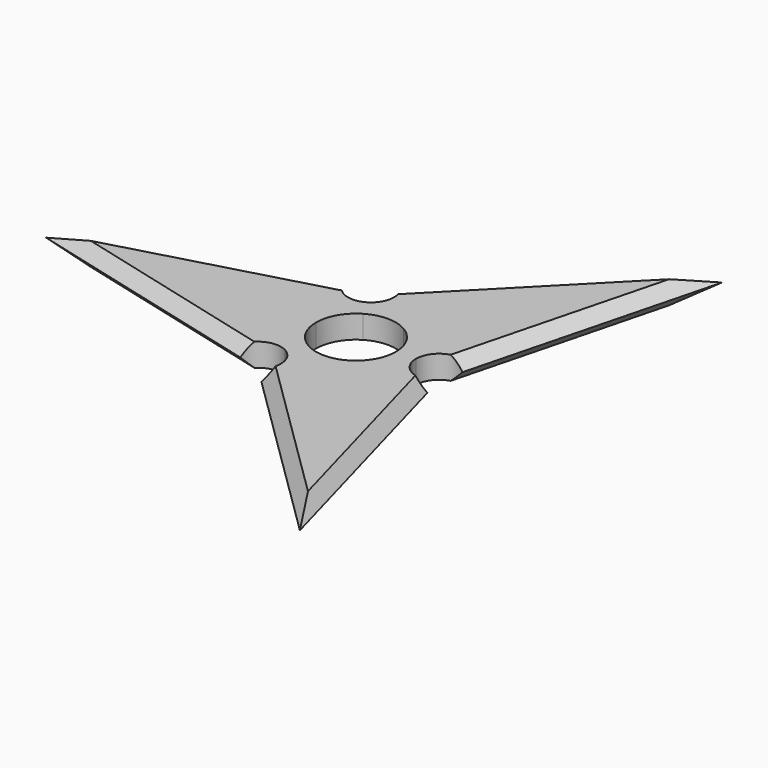
from build123d import *

# Parameters (mm, degrees)
F1_DEPTH = 6.35
F2_SIZE  = 3.17499


# Not quite as in the source:
# - a fillet or chamfer is up to 0.001 mm smaller than in the source, because OpenCascade refuses the exact size


with BuildPart() as f1:
    # F0 (on Top) → F1 (new body)
    with BuildSketch(Plane.XY):
        with BuildLine():
            Line((-17.3524573698, -16.6459077914), (19.1028173324, 47.7399711053))
            Line((19.1028173324, 47.7399711053), (-29.8718068032, -2.0647344031))
            ThreePointArc((-29.8718068032, -2.0647344031), (-28.46767213, -4.137767395), (-27.974045361, -6.5924349039))
            ThreePointArc((-27.974045361, -6.5924349039), (-28.8114925566, -9.7443012682), (-31.1029466457, -12.0648222317))
            Line((-31.1029466457, -12.0648222317), (-28.352068997, -16.7383418336))
            ThreePointArc((-28.352068997, -16.7383418336), (-22.8646469969, -15.2184562862), (-17.3524573698, -16.6459077914))
        make_face()
        with BuildLine():
            ThreePointArc((-31.1029466457, -12.0648222317), (-36.70470147, -12.4792826589), (-40.4436473061, -8.2874192794))
            Line((-40.4436473061, -8.2874192794), (-107.7592687025, -26.9322474098))
            Line((-107.7592687025, -26.9322474098), (-33.7718245819, -26.3105019555))
            ThreePointArc((-33.7718245819, -26.3105019555), (-32.3443730767, -20.7983123285), (-28.352068997, -16.7383418336))
            Line((-28.352068997, -16.7383418336), (-31.1029466457, -12.0648222317))
        make_face()
        with BuildLine():
            Line((-33.7718245819, -26.3105019555), (-107.7592687025, -26.9322474098))
            Line((-107.7592687025, -26.9322474098), (-40.1398164365, -44.4431632978))
            ThreePointArc((-40.1398164365, -44.4431632978), (-36.4718453922, -40.1890566965), (-30.8639164155, -40.5093177627))
            Line((-30.8639164155, -40.5093177627), (-28.1919685396, -35.7902280353))
            ThreePointArc((-28.1919685396, -35.7902280353), (-32.2519390345, -31.7979239556), (-33.7718245819, -26.3105019555))
        make_face()
        with BuildLine():
            Line((20.339812506, -99.4619274356), (-17.1923569125, -35.6977939932))
            ThreePointArc((-17.1923569125, -35.6977939932), (-22.6797789126, -37.2176795405), (-28.1919685396, -35.7902280353))
            Line((-28.1919685396, -35.7902280353), (-30.8639164155, -40.5093177627))
            ThreePointArc((-30.8639164155, -40.5093177627), (-28.5067207601, -42.8369871561), (-27.6425935032, -46.0350647422))
            ThreePointArc((-27.6425935032, -46.0350647422), (-28.1158002373, -48.440433926), (-29.4648930024, -50.4873033))
            Line((-29.4648930024, -50.4873033), (20.339812506, -99.4619274356))
        make_face()
        with BuildLine():
            ThreePointArc((1.6949843755, -32.1463060392), (-3.8231655338, -31.0968032352), (-6.3497758029, -26.0800637457))
            Line((-6.3497758029, -26.0800637457), (-11.7726013276, -26.1256338712))
            ThreePointArc((-11.7726013276, -26.1256338712), (-11.7723100484, -26.1718504844), (-11.7722129547, -26.2180679134))
            ThreePointArc((-11.7722129547, -26.2180679134), (-13.2229088841, -31.6779938989), (-17.1923569125, -35.6977939932))
            Line((-17.1923569125, -35.6977939932), (20.339812506, -99.4619274356))
            Line((20.339812506, -99.4619274356), (1.6949843755, -32.1463060392))
        make_face()
        with BuildLine():
            Line((1.5919014444, -19.8794811608), (19.1028173324, 47.7399711053))
            Line((19.1028173324, 47.7399711053), (-17.3524573698, -16.6459077914))
            ThreePointArc((-17.3524573698, -16.6459077914), (-13.2924868749, -20.6382118711), (-11.7726013276, -26.1256338712))
            Line((-11.7726013276, -26.1256338712), (-6.3497758029, -26.0800637457))
            ThreePointArc((-6.3497758029, -26.0800637457), (-3.9078316495, -21.0215715485), (1.5919014444, -19.8794811608))
        make_face()
    extrude(amount=F1_DEPTH)

    # F2 (size 3.175 in the source; OpenCascade refuses exactly that, so slightly less here)
    f2_edges = [f1.edges().sort_by_distance(p)[0] for p in [
        (-74.101458, -17.609833, 6.35),
        (-73.949543, -35.687705, 6.35),
        (-73.949543, -35.687705, 0),
        (-4.56254, -74.974615, 6.35),
        (11.017398, -65.804117, 6.35),
        (-5.384495, 22.837618, 6.35),
        (-74.101458, -17.609833, 0),
        (-4.56254, -74.974615, 0),
        (11.017398, -65.804117, 0),
        (-5.384495, 22.837618, 0),
        (10.347359, 13.930245, 0),
        (10.347359, 13.930245, 6.35),
    ]]
    chamfer(f2_edges, length=F2_SIZE)


solid = f1.part
